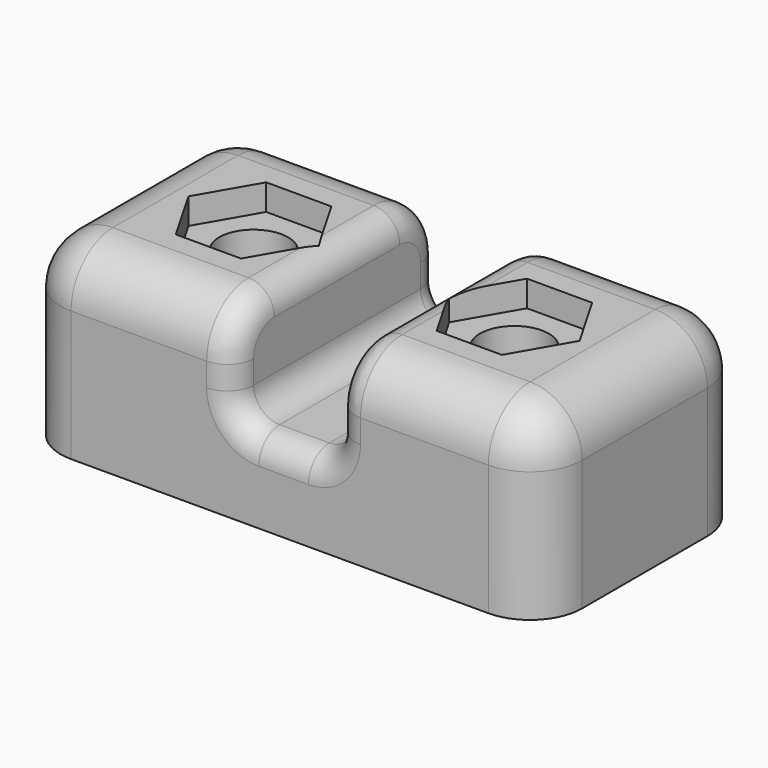
from build123d import *

# Parameters (mm, degrees)
F0_W         = 50.8
F0_H         = 25.4
F0_R         = 3.3655
F1_DEPTH     = 17.78
F2_W         = 9.906
F2_H         = 25.4
F3_DEPTH     = 9.906
F5_DEPTH     = 2.54
F6_R         = 5.08
F7_T1_DEPTH  = 25.4
F7_T3_DEPTH  = 4.826
F7_T5_DEPTH  = 15.24
F7_T7_DEPTH  = 2.286
F7_T10_ANGLE = 90
F7_T12_ANGLE = 90
F7_T14_ANGLE = 90
F7_T16_ANGLE = 90
F7_T18_ANGLE = 90
F7_T20_ANGLE = 90
F7_T22_ANGLE = 90
F7_T24_ANGLE = 90


# Not quite as in the source:
# - a fillet or chamfer that OpenCascade refuses, or shapes differently, is made with other operations: its cross-section is extruded or revolved along the edge and cut away or added
# - a feature names something its author has since deleted; it is built from what else it names


with BuildPart() as f1:
    # F0 (on Top) → F1 (new body)
    with BuildSketch(Plane.XY):
        with Locations((20.1624472324, -3.7984256737)):
            Rectangle(F0_W, F0_H)
        with Locations((7.4624472324, -3.7984256737)):
            Circle(F0_R, mode=Mode.SUBTRACT)
        with Locations((32.8624472324, -3.7984256737)):
            Circle(F0_R, mode=Mode.SUBTRACT)
    extrude(amount=F1_DEPTH)

    # F2 (on face) → F3 (cut)
    with BuildSketch(Plane.XY.offset(17.78)):
        with Locations((20.5434472324, -3.7984256737)):
            Rectangle(F2_W, F2_H)
    extrude(amount=-F3_DEPTH, mode=Mode.SUBTRACT)

    # F4 (on face) → F5 (cut)
    with BuildSketch(Plane.XY.offset(17.78)):
        Polygon((29.6874472324, -9.2976869878), (36.0374472324, -9.2976869878), (39.2124472324, -3.7984256737), (36.0374472324, 1.7008356403), (29.6874472324, 1.7008356403), (26.5124472324, -3.7984256737), align=None)
        Polygon((4.2874472324, -9.2976869878), (10.6374472324, -9.2976869878), (13.8124472324, -3.7984256737), (10.6374472324, 1.7008356403), (4.2874472324, 1.7008356403), (1.1124472324, -3.7984256737), align=None)
    extrude(amount=-F5_DEPTH, mode=Mode.SUBTRACT)

    # F6
    f6_edges = [f1.edges().sort_by_distance(p)[0] for p in [
        (45.562447, -3.798426, 17.78),
        (5.176447, 8.901574, 17.78),
        (-5.237553, -3.798426, 17.78),
        (5.176447, -16.498426, 17.78),
        (35.529447, -16.498426, 17.78),
        (35.529447, 8.901574, 17.78),
        (-5.237553, 8.901574, 8.89),
        (-5.237553, -16.498426, 8.89),
        (45.562447, -16.498426, 8.89),
        (45.562447, 8.901574, 8.89),
    ]]
    fillet(f6_edges, radius=F6_R)

    # F7: fillet of radius 2.54 on 10 edges, made by hand

    # F7_s2 → F7_t1 (join)
    with BuildSketch(Plane.XZ.offset(-8.9015743263)):
        with BuildLine():
            ThreePointArc((15.5904472324, 10.414), (16.3343960082, 8.6179487758), (18.1304472324, 7.874))
            Line((18.1304472324, 7.874), (15.5904472324, 7.874))
            Line((15.5904472324, 7.874), (15.5904472324, 10.414))
        make_face()
        with BuildLine():
            ThreePointArc((25.4964472324, 10.414), (24.7524984566, 8.6179487758), (22.9564472324, 7.874))
            Line((22.9564472324, 7.874), (25.4964472324, 7.874))
            Line((25.4964472324, 7.874), (25.4964472324, 10.414))
        make_face()
    extrude(amount=F7_T1_DEPTH)

    # F7_s4 → F7_t3 (cut)
    with BuildSketch(Plane.YZ.offset(18.1304472324)):
        with BuildLine():
            ThreePointArc((6.3615743263, 7.874), (8.1576255505, 7.1300512242), (8.9015743263, 5.334))
            Line((8.9015743263, 5.334), (8.9015743263, 7.874))
            Line((8.9015743263, 7.874), (6.3615743263, 7.874))
        make_face()
        with BuildLine():
            ThreePointArc((-16.4984256737, 5.334), (-15.7544768979, 7.1300512242), (-13.9584256737, 7.874))
            Line((-13.9584256737, 7.874), (-16.4984256737, 7.874))
            Line((-16.4984256737, 7.874), (-16.4984256737, 5.334))
        make_face()
    extrude(amount=F7_T3_DEPTH, mode=Mode.SUBTRACT)

    # F7_s6 → F7_t5 (cut)
    with BuildSketch(Plane.XZ.offset(-3.8215743263)):
        with BuildLine():
            ThreePointArc((15.5904472324, 15.24), (14.8464984566, 17.0360512242), (13.0504472324, 17.78))
            Line((13.0504472324, 17.78), (15.5904472324, 17.78))
            Line((15.5904472324, 17.78), (15.5904472324, 15.24))
        make_face()
        with BuildLine():
            ThreePointArc((25.4964472324, 15.24), (26.2403960082, 17.0360512242), (28.0364472324, 17.78))
            Line((28.0364472324, 17.78), (25.4964472324, 17.78))
            Line((25.4964472324, 17.78), (25.4964472324, 15.24))
        make_face()
    extrude(amount=F7_T5_DEPTH, mode=Mode.SUBTRACT)

    # F7_s8 → F7_t7 (cut)
    with BuildSketch(Plane.XY.offset(10.414)):
        with BuildLine():
            ThreePointArc((25.4964472324, 6.3615743263), (26.2403960082, 8.1576255505), (28.0364472324, 8.9015743263))
            Line((28.0364472324, 8.9015743263), (25.4964472324, 8.9015743263))
            Line((25.4964472324, 8.9015743263), (25.4964472324, 6.3615743263))
        make_face()
        with BuildLine():
            ThreePointArc((15.5904472324, 6.3615743263), (14.8464984566, 8.1576255505), (13.0504472324, 8.9015743263))
            Line((13.0504472324, 8.9015743263), (15.5904472324, 8.9015743263))
            Line((15.5904472324, 8.9015743263), (15.5904472324, 6.3615743263))
        make_face()
        with BuildLine():
            ThreePointArc((28.0364472324, -16.4984256737), (26.2403960082, -15.7544768979), (25.4964472324, -13.9584256737))
            Line((25.4964472324, -13.9584256737), (25.4964472324, -16.4984256737))
            Line((25.4964472324, -16.4984256737), (28.0364472324, -16.4984256737))
        make_face()
        with BuildLine():
            ThreePointArc((13.0504472324, -16.4984256737), (14.8464984566, -15.7544768979), (15.5904472324, -13.9584256737))
            Line((15.5904472324, -13.9584256737), (15.5904472324, -16.4984256737))
            Line((15.5904472324, -16.4984256737), (13.0504472324, -16.4984256737))
        make_face()
    extrude(amount=F7_T7_DEPTH, mode=Mode.SUBTRACT)

    # F7_s9 → F7_t10 (revolve, cut)
    with BuildSketch(Plane.XY.offset(12.7)):
        with BuildLine():
            ThreePointArc((13.0504472324, -16.4984256737), (14.8464984566, -15.7544768979), (15.5904472324, -13.9584256737))
            Line((15.5904472324, -13.9584256737), (15.5904472324, -16.4984256737))
            Line((15.5904472324, -16.4984256737), (13.0504472324, -16.4984256737))
        make_face()
    revolve(axis=Axis((15.5904472324, -11.4184256737, 12.7), (-1, 0, 0)), revolution_arc=F7_T10_ANGLE, mode=Mode.SUBTRACT)

    # F7_s11 → F7_t12 (revolve, cut)
    with BuildSketch(Plane.XY.offset(12.7)):
        with BuildLine():
            ThreePointArc((28.0364472324, -16.4984256737), (26.2403960082, -15.7544768979), (25.4964472324, -13.9584256737))
            Line((25.4964472324, -13.9584256737), (25.4964472324, -16.4984256737))
            Line((25.4964472324, -16.4984256737), (28.0364472324, -16.4984256737))
        make_face()
    revolve(axis=Axis((25.4964472324, -11.4184256737, 12.7), (-1, 0, 0)), revolution_arc=F7_T12_ANGLE, mode=Mode.SUBTRACT)

    # F7_s13 → F7_t14 (revolve, cut)
    with BuildSketch(Plane.XZ.offset(-3.8215743263)):
        with BuildLine():
            ThreePointArc((15.5904472324, 15.24), (14.8464984566, 17.0360512242), (13.0504472324, 17.78))
            Line((13.0504472324, 17.78), (15.5904472324, 17.78))
            Line((15.5904472324, 17.78), (15.5904472324, 15.24))
        make_face()
    revolve(axis=Axis((15.5904472324, 3.8215743263, 12.7), (-1, 0, 0)), revolution_arc=F7_T14_ANGLE, mode=Mode.SUBTRACT)

    # F7_s15 → F7_t16 (revolve, cut)
    with BuildSketch(Plane.XZ.offset(-3.8215743263)):
        with BuildLine():
            ThreePointArc((25.4964472324, 15.24), (26.2403960082, 17.0360512242), (28.0364472324, 17.78))
            Line((28.0364472324, 17.78), (25.4964472324, 17.78))
            Line((25.4964472324, 17.78), (25.4964472324, 15.24))
        make_face()
    revolve(axis=Axis((25.4964472324, 3.8215743263, 12.7), (-1, 0, 0)), revolution_arc=F7_T16_ANGLE, mode=Mode.SUBTRACT)

    # F7_s17 → F7_t18 (revolve, cut)
    with BuildSketch(Plane.XY.offset(10.414)):
        with BuildLine():
            ThreePointArc((13.0504472324, -16.4984256737), (14.8464984566, -15.7544768979), (15.5904472324, -13.9584256737))
            Line((15.5904472324, -13.9584256737), (15.5904472324, -16.4984256737))
            Line((15.5904472324, -16.4984256737), (13.0504472324, -16.4984256737))
        make_face()
    revolve(axis=Axis((18.1304472324, -16.4984256737, 10.414), (0, -1, 0)), revolution_arc=F7_T18_ANGLE, mode=Mode.SUBTRACT)

    # F7_s19 → F7_t20 (revolve, cut)
    with BuildSketch(Plane.XY.offset(10.414)):
        with BuildLine():
            ThreePointArc((28.0364472324, -16.4984256737), (26.2403960082, -15.7544768979), (25.4964472324, -13.9584256737))
            Line((25.4964472324, -13.9584256737), (25.4964472324, -16.4984256737))
            Line((25.4964472324, -16.4984256737), (28.0364472324, -16.4984256737))
        make_face()
    revolve(axis=Axis((22.9564472324, -16.4984256737, 10.414), (0, 1, 0)), revolution_arc=F7_T20_ANGLE, mode=Mode.SUBTRACT)

    # F7_s21 → F7_t22 (revolve, cut)
    with BuildSketch(Plane.XY.offset(10.414)):
        with BuildLine():
            ThreePointArc((13.0504472324, 8.9015743263), (14.8464984566, 8.1576255505), (15.5904472324, 6.3615743263))
            Line((15.5904472324, 6.3615743263), (15.5904472324, 8.9015743263))
            Line((15.5904472324, 8.9015743263), (13.0504472324, 8.9015743263))
        make_face()
    revolve(axis=Axis((18.1304472324, 8.9015743263, 10.414), (0, -1, 0)), revolution_arc=F7_T22_ANGLE, mode=Mode.SUBTRACT)

    # F7_s23 → F7_t24 (revolve, cut)
    with BuildSketch(Plane.XY.offset(10.414)):
        with BuildLine():
            ThreePointArc((28.0364472324, 8.9015743263), (26.2403960082, 8.1576255505), (25.4964472324, 6.3615743263))
            Line((25.4964472324, 6.3615743263), (25.4964472324, 8.9015743263))
            Line((25.4964472324, 8.9015743263), (28.0364472324, 8.9015743263))
        make_face()
    revolve(axis=Axis((22.9564472324, 8.9015743263, 10.414), (0, 1, 0)), revolution_arc=F7_T24_ANGLE, mode=Mode.SUBTRACT)


solid = f1.part
